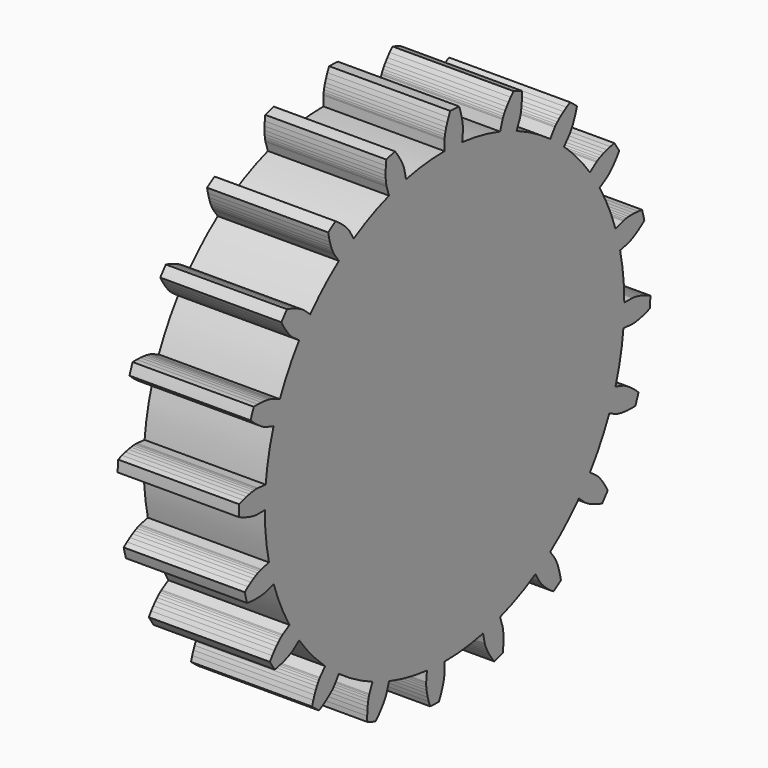
from build123d import *

# Parameters (mm, degrees)
F2_DEPTH = 12.7


# Not quite as in the source:
# - a variable given as a bare number and used for a length is read in inches; the dataset says mm whatever the document's units were


with BuildPart() as f2:
    # F1 (on Right) → F2 (new body)
    with BuildSketch(Plane.YZ):
        with BuildLine():
            ThreePointArc((23.4497989506, -2.3096036071), (23.5348795184, -1.1561944904), (23.5632625, 0))
            ThreePointArc((23.5632625, 0), (23.4259947642, 2.5397064696), (23.0157908626, 5.0498228298))
            ThreePointArc((23.0157908626, 5.0498228298), (22.7402842725, 6.1730714275), (22.4099943458, 7.2814485554))
            ThreePointArc((22.4099943458, 7.2814485554), (21.4946325114, 9.6544348796), (20.3288368046, 11.914937424))
            ThreePointArc((20.3288368046, 11.914937424), (19.7197115612, 12.8980741038), (19.0630798054, 13.8501381934))
            ThreePointArc((19.0630798054, 13.8501381934), (17.4592258664, 15.8241199373), (15.6519545608, 17.6137349268))
            ThreePointArc((15.6519545608, 17.6137349268), (14.7688360869, 18.3605234207), (13.8501381934, 19.0630798054))
            ThreePointArc((13.8501381934, 19.0630798054), (11.7147885481, 20.4448298823), (9.442949951, 21.5883773329))
            ThreePointArc((9.442949951, 21.5883773329), (8.372284036, 22.0257167798), (7.2814485554, 22.4099943458))
            ThreePointArc((7.2814485554, 22.4099943458), (4.8236261049, 23.064257431), (2.3096036071, 23.4497989506))
            ThreePointArc((2.3096036071, 23.4497989506), (1.1561944904, 23.5348795184), (0, 23.5632625))
            ThreePointArc((0, 23.5632625), (-2.5397064696, 23.4259947642), (-5.0498228298, 23.0157908626))
            ThreePointArc((-5.0498228298, 23.0157908626), (-6.1730714275, 22.7402842725), (-7.2814485554, 22.4099943458))
            ThreePointArc((-7.2814485554, 22.4099943458), (-9.6544348796, 21.4946325114), (-11.914937424, 20.3288368046))
            ThreePointArc((-11.914937424, 20.3288368046), (-12.8980741038, 19.7197115612), (-13.8501381934, 19.0630798054))
            ThreePointArc((-13.8501381934, 19.0630798054), (-15.8241199373, 17.4592258664), (-17.6137349268, 15.6519545608))
            ThreePointArc((-17.6137349268, 15.6519545608), (-18.3605234207, 14.7688360869), (-19.0630798054, 13.8501381934))
            ThreePointArc((-19.0630798054, 13.8501381934), (-20.4448298823, 11.7147885481), (-21.5883773329, 9.442949951))
            ThreePointArc((-21.5883773329, 9.442949951), (-22.0257167798, 8.372284036), (-22.4099943458, 7.2814485554))
            ThreePointArc((-22.4099943458, 7.2814485554), (-23.064257431, 4.8236261049), (-23.4497989506, 2.3096036071))
            ThreePointArc((-23.4497989506, 2.3096036071), (-23.5348795184, 1.1561944904), (-23.5632625, 0))
            ThreePointArc((-23.5632625, 0), (-23.4259947642, -2.5397064696), (-23.0157908626, -5.0498228298))
            ThreePointArc((-23.0157908626, -5.0498228298), (-22.7402842725, -6.1730714275), (-22.4099943458, -7.2814485554))
            ThreePointArc((-22.4099943458, -7.2814485554), (-21.4946325114, -9.6544348796), (-20.3288368046, -11.914937424))
            ThreePointArc((-20.3288368046, -11.914937424), (-19.7197115612, -12.8980741038), (-19.0630798054, -13.8501381934))
            ThreePointArc((-19.0630798054, -13.8501381934), (-17.4592258664, -15.8241199373), (-15.6519545608, -17.6137349268))
            ThreePointArc((-15.6519545608, -17.6137349268), (-14.7688360869, -18.3605234207), (-13.8501381934, -19.0630798054))
            ThreePointArc((-13.8501381934, -19.0630798054), (-11.7147885481, -20.4448298823), (-9.442949951, -21.5883773329))
            ThreePointArc((-9.442949951, -21.5883773329), (-8.372284036, -22.0257167798), (-7.2814485554, -22.4099943458))
            ThreePointArc((-7.2814485554, -22.4099943458), (-4.8236261049, -23.064257431), (-2.3096036071, -23.4497989506))
            ThreePointArc((-2.3096036071, -23.4497989506), (-1.1561944904, -23.5348795184), (0, -23.5632625))
            ThreePointArc((0, -23.5632625), (2.5397064696, -23.4259947642), (5.0498228298, -23.0157908626))
            ThreePointArc((5.0498228298, -23.0157908626), (6.1730714275, -22.7402842725), (7.2814485554, -22.4099943458))
            ThreePointArc((7.2814485554, -22.4099943458), (9.6544348796, -21.4946325114), (11.914937424, -20.3288368046))
            ThreePointArc((11.914937424, -20.3288368046), (12.8980741038, -19.7197115612), (13.8501381934, -19.0630798054))
            ThreePointArc((13.8501381934, -19.0630798054), (15.8241199373, -17.4592258664), (17.6137349268, -15.6519545608))
            ThreePointArc((17.6137349268, -15.6519545608), (18.3605234207, -14.7688360869), (19.0630798054, -13.8501381934))
            ThreePointArc((19.0630798054, -13.8501381934), (20.4448298823, -11.7147885481), (21.5883773329, -9.442949951))
            ThreePointArc((21.5883773329, -9.442949951), (22.0257167798, -8.372284036), (22.4099943458, -7.2814485554))
            ThreePointArc((22.4099943458, -7.2814485554), (23.064257431, -4.8236261049), (23.4497989506, -2.3096036071))
        make_face()
        with BuildLine():
            Line((-23.3873833018, -7.5990214781), (-22.4099943458, -7.2814485554))
            ThreePointArc((-22.4099943458, -7.2814485554), (-22.7402842725, -6.1730714275), (-23.0157908626, -5.0498228298))
            Line((-23.0157908626, -5.0498228298), (-24.0196010133, -5.2700656816))
            Line((-24.0196010133, -5.2700656816), (-24.0493872246, -5.2776496958))
            Line((-24.0493872246, -5.2776496958), (-24.1376440155, -5.3043486651))
            Line((-24.1376440155, -5.3043486651), (-24.2823879504, -5.3559820874))
            Line((-24.2823879504, -5.3559820874), (-24.4812024195, -5.4382116757))
            Line((-24.4812024195, -5.4382116757), (-24.7312488149, -5.5565127334))
            Line((-24.7312488149, -5.5565127334), (-25.0292794786, -5.7161462693))
            Line((-25.0292794786, -5.7161462693), (-25.3716523755, -5.9221319592))
            Line((-25.3716523755, -5.9221319592), (-25.7543474377, -6.1792220552))
            Line((-25.7543474377, -6.1792220552), (-26.1729845215, -6.491876343))
            Line((-26.1729845215, -6.491876343), (-26.1912910496, -6.5070292303))
            ThreePointArc((-26.1912910496, -6.5070292303), (-26.0449257315, -7.0701485055), (-25.8864547108, -7.6299815699))
            Line((-25.8864547108, -7.6299815699), (-25.8629988703, -7.633797656))
            Line((-25.8629988703, -7.633797656), (-25.3437303169, -7.6918483328))
            Line((-25.3437303169, -7.6918483328), (-24.8835666247, -7.720136219))
            Line((-24.8835666247, -7.720136219), (-24.4840315708, -7.7247237769))
            Line((-24.4840315708, -7.7247237769), (-24.1461903947, -7.7117437148))
            Line((-24.1461903947, -7.7117437148), (-23.8706469692, -7.6873683017))
            Line((-23.8706469692, -7.6873683017), (-23.6575428926, -7.6577785929))
            Line((-23.6575428926, -7.6577785929), (-23.5065585022, -7.6291336838))
            Line((-23.5065585022, -7.6291336838), (-23.4169158032, -7.6075401056))
            Line((-23.4169158032, -7.6075401056), (-23.3873833018, -7.5990214781))
        make_face()
        with BuildLine():
            Line((-19.8944965109, -14.4541977884), (-19.0630798054, -13.8501381934))
            ThreePointArc((-19.0630798054, -13.8501381934), (-19.7197115612, -12.8980741038), (-20.3288368046, -11.914937424))
            Line((-20.3288368046, -11.914937424), (-21.2154582055, -12.434595219))
            Line((-21.2154582055, -12.434595219), (-21.2414429865, -12.4510124906))
            Line((-21.2414429865, -12.4510124906), (-21.3171297473, -12.5036775676))
            Line((-21.3171297473, -12.5036775676), (-21.4388338049, -12.5975122061))
            Line((-21.4388338049, -12.5975122061), (-21.602507261, -12.7371542416))
            Line((-21.602507261, -12.7371542416), (-21.8037584774, -12.9269338189))
            Line((-21.8037584774, -12.9269338189), (-22.0378730067, -13.1708508734))
            Line((-22.0378730067, -13.1708508734), (-22.2998359026, -13.4725539495))
            Line((-22.2998359026, -13.4725539495), (-22.5843553265, -13.8353204385))
            Line((-22.5843553265, -13.8353204385), (-22.8858873647, -14.2620383097))
            Line((-22.8858873647, -14.2620383097), (-22.8986154078, -14.2821065902))
            ThreePointArc((-22.8986154078, -14.2821065902), (-22.5854002924, -14.7724354756), (-22.2616874646, -15.2558981211))
            Line((-22.2616874646, -15.255898121), (-22.2382003992, -15.2522791813))
            Line((-22.2382003992, -15.2522791813), (-21.7264080121, -15.147025848))
            Line((-21.7264080121, -15.147025848), (-21.2800248965, -15.0317308255))
            Line((-21.2800248965, -15.0317308255), (-20.8986268467, -14.9126307308))
            Line((-20.8986268467, -14.9126307308), (-20.5813318544, -14.7958872934))
            Line((-20.5813318544, -14.7958872934), (-20.326806901, -14.6875572967))
            Line((-20.326806901, -14.6875572967), (-20.1332766032, -14.5935630301))
            Line((-20.1332766032, -14.5935630301), (-19.9985336785, -14.5196633601))
            Line((-19.9985336785, -14.5196633601), (-19.9199511881, -14.4714255295))
            Line((-19.9199511881, -14.4714255295), (-19.8944965109, -14.4541977884))
        make_face()
        with BuildLine():
            Line((-14.4541977884, -19.8944965109), (-13.8501381934, -19.0630798054))
            ThreePointArc((-13.8501381934, -19.0630798054), (-14.7688360869, -18.3605234207), (-15.6519545608, -17.6137349268))
            Line((-15.6519545608, -17.6137349268), (-16.3345985316, -18.3819399395))
            Line((-16.3345985316, -18.3819399395), (-16.3542383111, -18.4055834316))
            Line((-16.3542383111, -18.4055834316), (-16.4099462943, -18.4790593916))
            Line((-16.4099462943, -18.4790593916), (-16.4966972334, -18.605910058))
            Line((-16.4966972334, -18.605910058), (-16.6092081783, -18.7892954052))
            Line((-16.6092081783, -18.7892954052), (-16.7419643445, -19.031976555))
            Line((-16.7419643445, -19.031976555), (-16.8892459781, -19.3363008272))
            Line((-16.8892459781, -19.3363008272), (-17.0451561195, -19.7041884905))
            Line((-17.0451561195, -19.7041884905), (-17.2036491615, -20.137121261))
            Line((-17.2036491615, -20.137121261), (-17.3585600973, -20.6361325971))
            Line((-17.3585600973, -20.6361325971), (-17.3644637459, -20.6591518477))
            ThreePointArc((-17.3644637459, -20.6591518477), (-16.915058511, -21.0286935358), (-16.457791143, -21.38846107))
            Line((-16.457791143, -21.38846107), (-16.4365719304, -21.3777613514))
            Line((-16.4365719304, -21.3777613514), (-15.9823535143, -21.1195069377))
            Line((-15.9823535143, -21.1195069377), (-15.5934460648, -20.8719148865))
            Line((-15.5934460648, -20.8719148865), (-15.2675189175, -20.6407854863))
            Line((-15.2675189175, -20.6407854863), (-15.0018291537, -20.4317063346))
            Line((-15.0018291537, -20.4317063346), (-14.7932373481, -20.2500258493))
            Line((-14.7932373481, -20.2500258493), (-14.6382249231, -20.1008278386))
            Line((-14.6382249231, -20.1008278386), (-14.5329130404, -19.9889072223))
            Line((-14.5329130404, -19.9889072223), (-14.4730829603, -19.9187469941))
            Line((-14.4730829603, -19.9187469941), (-14.4541977884, -19.8944965109))
        make_face()
        with BuildLine():
            Line((-7.5990214781, -23.3873833018), (-7.2814485554, -22.4099943458))
            ThreePointArc((-7.2814485554, -22.4099943458), (-8.372284036, -22.0257167798), (-9.442949951, -21.5883773329))
            Line((-9.442949951, -21.5883773329), (-9.8547945437, -22.5299323042))
            Line((-9.8547945437, -22.5299323042), (-9.866166843, -22.558487627))
            Line((-9.866166843, -22.558487627), (-9.8964429632, -22.6455821311))
            Line((-9.8964429632, -22.6455821311), (-9.9397489974, -22.7930317984))
            Line((-9.9397489974, -22.7930317984), (-9.9900840759, -23.0022094219))
            Line((-9.9900840759, -23.0022094219), (-10.0413500933, -23.2740368222))
            Line((-10.0413500933, -23.2740368222), (-10.0873818788, -23.6089789322))
            Line((-10.0873818788, -23.6089789322), (-10.1219776947, -24.0070397749))
            Line((-10.1219776947, -24.0070397749), (-10.1389299516, -24.4677603508))
            Line((-10.1389299516, -24.4677603508), (-10.1320560234, -24.9902184456))
            Line((-10.1320560234, -24.9902184456), (-10.1305573872, -25.0139353816))
            ThreePointArc((-10.1305573872, -25.0139353816), (-9.5889529483, -25.2265165571), (-9.0428915563, -25.4273724272))
            Line((-9.0428915563, -25.4273724272), (-9.0260172807, -25.4106392928))
            Line((-9.0260172807, -25.4106392928), (-8.6738348989, -25.0246635401))
            Line((-8.6738348989, -25.0246635401), (-8.3804720864, -24.6690104953))
            Line((-8.3804720864, -24.6690104953), (-8.1419198617, -24.3484763457))
            Line((-8.1419198617, -24.3484763457), (-7.9538428915, -24.0675276037))
            Line((-7.9538428915, -24.0675276037), (-7.8116026531, -23.8302807815))
            Line((-7.8116026531, -23.8302807815), (-7.710281797, -23.6404835675))
            Line((-7.710281797, -23.6404835675), (-7.6447096172, -23.5014975746))
            Line((-7.6447096172, -23.5014975746), (-7.6094885324, -23.4162827209))
            Line((-7.6094885324, -23.4162827209), (-7.5990214781, -23.3873833018))
        make_face()
        with BuildLine():
            Line((0, -24.5909500656), (0, -23.5632625))
            ThreePointArc((0, -23.5632625), (-1.1561944904, -23.5348795184), (-2.3096036071, -23.4497989506))
            Line((-2.3096036071, -23.4497989506), (-2.4103346034, -24.4725379196))
            Line((-2.4103346034, -24.4725379196), (-2.4123262228, -24.5032098793))
            Line((-2.4123262228, -24.5032098793), (-2.4142068423, -24.5953975106))
            Line((-2.4142068423, -24.5953975106), (-2.4098288753, -24.749012778))
            Line((-2.4098288753, -24.749012778), (-2.3930609392, -24.9635069146))
            Line((-2.3930609392, -24.9635069146), (-2.3578185329, -25.2378722056))
            Line((-2.3578185329, -25.2378722056), (-2.2980945583, -25.5706456859))
            Line((-2.2980945583, -25.5706456859), (-2.2079895693, -25.9599147393))
            Line((-2.2079895693, -25.9599147393), (-2.0817416361, -26.4033245806))
            Line((-2.0817416361, -26.4033245806), (-1.9137557117, -26.8980875955))
            Line((-1.9137557117, -26.8980875955), (-1.9050014877, -26.920180638))
            ThreePointArc((-1.9050014877, -26.920180638), (-1.3242138609, -26.9549923743), (-0.7428107384, -26.9772754083))
            Line((-0.7428107384, -26.9772754083), (-0.7319331716, -26.9561468139))
            Line((-0.7319331716, -26.9561468139), (-0.5162608895, -26.4802317181))
            Line((-0.5162608895, -26.4802317181), (-0.3471591099, -26.0513314777))
            Line((-0.3471591099, -26.0513314777), (-0.2193329616, -25.6727686945))
            Line((-0.2193329616, -25.6727686945), (-0.1272790694, -25.3474515827))
            Line((-0.1272790694, -25.3474515827), (-0.0653138637, -25.0778617955))
            Line((-0.0653138637, -25.0778617955), (-0.0276025679, -24.8660440519))
            Line((-0.0276025679, -24.8660440519), (-0.0081887528, -24.7135975998))
            Line((-0.0081887528, -24.7135975998), (-0.0010243486, -24.6216695442))
            Line((-0.0010243486, -24.6216695442), (0, -24.5909500656))
        make_face()
        with BuildLine():
            Line((7.5990214781, -23.3873833018), (7.2814485554, -22.4099943458))
            ThreePointArc((7.2814485554, -22.4099943458), (6.1730714275, -22.7402842725), (5.0498228298, -23.0157908626))
            Line((5.0498228298, -23.0157908626), (5.2700656816, -24.0196010133))
            Line((5.2700656816, -24.0196010133), (5.2776496958, -24.0493872246))
            Line((5.2776496958, -24.0493872246), (5.3043486651, -24.1376440155))
            Line((5.3043486651, -24.1376440155), (5.3559820874, -24.2823879504))
            Line((5.3559820874, -24.2823879504), (5.4382116757, -24.4812024195))
            Line((5.4382116757, -24.4812024195), (5.5565127334, -24.7312488149))
            Line((5.5565127334, -24.7312488149), (5.7161462693, -25.0292794786))
            Line((5.7161462693, -25.0292794786), (5.9221319592, -25.3716523755))
            Line((5.9221319592, -25.3716523755), (6.1792220552, -25.7543474377))
            Line((6.1792220552, -25.7543474377), (6.491876343, -26.1729845215))
            Line((6.491876343, -26.1729845215), (6.5070292303, -26.1912910496))
            ThreePointArc((6.5070292303, -26.1912910496), (7.0701485055, -26.0449257315), (7.6299815699, -25.8864547108))
            Line((7.6299815699, -25.8864547108), (7.633797656, -25.8629988703))
            Line((7.633797656, -25.8629988703), (7.6918483328, -25.3437303169))
            Line((7.6918483328, -25.3437303169), (7.720136219, -24.8835666247))
            Line((7.720136219, -24.8835666247), (7.7247237769, -24.4840315708))
            Line((7.7247237769, -24.4840315708), (7.7117437148, -24.1461903947))
            Line((7.7117437148, -24.1461903947), (7.6873683017, -23.8706469692))
            Line((7.6873683017, -23.8706469692), (7.6577785929, -23.6575428926))
            Line((7.6577785929, -23.6575428926), (7.6291336838, -23.5065585022))
            Line((7.6291336838, -23.5065585022), (7.6075401056, -23.4169158032))
            Line((7.6075401056, -23.4169158032), (7.5990214781, -23.3873833018))
        make_face()
        with BuildLine():
            Line((14.4541977884, -19.8944965109), (13.8501381934, -19.0630798054))
            ThreePointArc((13.8501381934, -19.0630798054), (12.8980741038, -19.7197115612), (11.914937424, -20.3288368046))
            Line((11.914937424, -20.3288368046), (12.434595219, -21.2154582055))
            Line((12.434595219, -21.2154582055), (12.4510124906, -21.2414429865))
            Line((12.4510124906, -21.2414429865), (12.5036775676, -21.3171297473))
            Line((12.5036775676, -21.3171297473), (12.5975122061, -21.4388338049))
            Line((12.5975122061, -21.4388338049), (12.7371542416, -21.602507261))
            Line((12.7371542416, -21.602507261), (12.9269338189, -21.8037584774))
            Line((12.9269338189, -21.8037584774), (13.1708508734, -22.0378730067))
            Line((13.1708508734, -22.0378730067), (13.4725539495, -22.2998359026))
            Line((13.4725539495, -22.2998359026), (13.8353204385, -22.5843553265))
            Line((13.8353204385, -22.5843553265), (14.2620383097, -22.8858873647))
            Line((14.2620383097, -22.8858873647), (14.2821065902, -22.8986154078))
            ThreePointArc((14.2821065902, -22.8986154078), (14.7724354756, -22.5854002924), (15.2558981211, -22.2616874646))
            Line((15.255898121, -22.2616874646), (15.2522791813, -22.2382003992))
            Line((15.2522791813, -22.2382003992), (15.147025848, -21.7264080121))
            Line((15.147025848, -21.7264080121), (15.0317308255, -21.2800248965))
            Line((15.0317308255, -21.2800248965), (14.9126307308, -20.8986268467))
            Line((14.9126307308, -20.8986268467), (14.7958872934, -20.5813318544))
            Line((14.7958872934, -20.5813318544), (14.6875572967, -20.326806901))
            Line((14.6875572967, -20.326806901), (14.5935630301, -20.1332766032))
            Line((14.5935630301, -20.1332766032), (14.5196633601, -19.9985336785))
            Line((14.5196633601, -19.9985336785), (14.4714255295, -19.9199511881))
            Line((14.4714255295, -19.9199511881), (14.4541977884, -19.8944965109))
        make_face()
        with BuildLine():
            Line((19.8944965109, -14.4541977884), (19.0630798054, -13.8501381934))
            ThreePointArc((19.0630798054, -13.8501381934), (18.3605234207, -14.7688360869), (17.6137349268, -15.6519545608))
            Line((17.6137349268, -15.6519545608), (18.3819399395, -16.3345985316))
            Line((18.3819399395, -16.3345985316), (18.4055834316, -16.3542383111))
            Line((18.4055834316, -16.3542383111), (18.4790593916, -16.4099462943))
            Line((18.4790593916, -16.4099462943), (18.605910058, -16.4966972334))
            Line((18.605910058, -16.4966972334), (18.7892954052, -16.6092081783))
            Line((18.7892954052, -16.6092081783), (19.031976555, -16.7419643445))
            Line((19.031976555, -16.7419643445), (19.3363008272, -16.8892459781))
            Line((19.3363008272, -16.8892459781), (19.7041884905, -17.0451561195))
            Line((19.7041884905, -17.0451561195), (20.137121261, -17.2036491615))
            Line((20.137121261, -17.2036491615), (20.6361325971, -17.3585600973))
            Line((20.6361325971, -17.3585600973), (20.6591518477, -17.3644637459))
            ThreePointArc((20.6591518477, -17.3644637459), (21.0286935358, -16.915058511), (21.38846107, -16.457791143))
            Line((21.38846107, -16.457791143), (21.3777613514, -16.4365719304))
            Line((21.3777613514, -16.4365719304), (21.1195069377, -15.9823535143))
            Line((21.1195069377, -15.9823535143), (20.8719148865, -15.5934460648))
            Line((20.8719148865, -15.5934460648), (20.6407854863, -15.2675189175))
            Line((20.6407854863, -15.2675189175), (20.4317063346, -15.0018291537))
            Line((20.4317063346, -15.0018291537), (20.2500258493, -14.7932373481))
            Line((20.2500258493, -14.7932373481), (20.1008278386, -14.6382249231))
            Line((20.1008278386, -14.6382249231), (19.9889072223, -14.5329130404))
            Line((19.9889072223, -14.5329130404), (19.9187469941, -14.4730829603))
            Line((19.9187469941, -14.4730829603), (19.8944965109, -14.4541977884))
        make_face()
        with BuildLine():
            Line((23.3873833018, -7.5990214781), (22.4099943458, -7.2814485554))
            ThreePointArc((22.4099943458, -7.2814485554), (22.0257167798, -8.372284036), (21.5883773329, -9.442949951))
            Line((21.5883773329, -9.442949951), (22.5299323042, -9.8547945437))
            Line((22.5299323042, -9.8547945437), (22.558487627, -9.866166843))
            Line((22.558487627, -9.866166843), (22.6455821311, -9.8964429632))
            Line((22.6455821311, -9.8964429632), (22.7930317984, -9.9397489974))
            Line((22.7930317984, -9.9397489974), (23.0022094219, -9.9900840759))
            Line((23.0022094219, -9.9900840759), (23.2740368222, -10.0413500933))
            Line((23.2740368222, -10.0413500933), (23.6089789322, -10.0873818788))
            Line((23.6089789322, -10.0873818788), (24.0070397749, -10.1219776947))
            Line((24.0070397749, -10.1219776947), (24.4677603508, -10.1389299516))
            Line((24.4677603508, -10.1389299516), (24.9902184456, -10.1320560234))
            Line((24.9902184456, -10.1320560234), (25.0139353816, -10.1305573872))
            ThreePointArc((25.0139353816, -10.1305573872), (25.2265165571, -9.5889529483), (25.4273724272, -9.0428915563))
            Line((25.4273724272, -9.0428915563), (25.4106392928, -9.0260172807))
            Line((25.4106392928, -9.0260172807), (25.0246635401, -8.6738348989))
            Line((25.0246635401, -8.6738348989), (24.6690104953, -8.3804720864))
            Line((24.6690104953, -8.3804720864), (24.3484763457, -8.1419198617))
            Line((24.3484763457, -8.1419198617), (24.0675276037, -7.9538428915))
            Line((24.0675276037, -7.9538428915), (23.8302807815, -7.8116026531))
            Line((23.8302807815, -7.8116026531), (23.6404835675, -7.710281797))
            Line((23.6404835675, -7.710281797), (23.5014975746, -7.6447096172))
            Line((23.5014975746, -7.6447096172), (23.4162827209, -7.6094885324))
            Line((23.4162827209, -7.6094885324), (23.3873833018, -7.5990214781))
        make_face()
        with BuildLine():
            Line((24.5909500656, 0), (23.5632625, 0))
            ThreePointArc((23.5632625, 0), (23.5348795184, -1.1561944904), (23.4497989506, -2.3096036071))
            Line((23.4497989506, -2.3096036071), (24.4725379196, -2.4103346034))
            Line((24.4725379196, -2.4103346034), (24.5032098793, -2.4123262228))
            Line((24.5032098793, -2.4123262228), (24.5953975106, -2.4142068423))
            Line((24.5953975106, -2.4142068423), (24.749012778, -2.4098288753))
            Line((24.749012778, -2.4098288753), (24.9635069146, -2.3930609392))
            Line((24.9635069146, -2.3930609392), (25.2378722056, -2.3578185329))
            Line((25.2378722056, -2.3578185329), (25.5706456859, -2.2980945583))
            Line((25.5706456859, -2.2980945583), (25.9599147393, -2.2079895693))
            Line((25.9599147393, -2.2079895693), (26.4033245806, -2.0817416361))
            Line((26.4033245806, -2.0817416361), (26.8980875955, -1.9137557117))
            Line((26.8980875955, -1.9137557117), (26.920180638, -1.9050014877))
            ThreePointArc((26.920180638, -1.9050014877), (26.9549923743, -1.3242138609), (26.9772754083, -0.7428107384))
            Line((26.9772754083, -0.7428107384), (26.9561468139, -0.7319331716))
            Line((26.9561468139, -0.7319331716), (26.4802317181, -0.5162608895))
            Line((26.4802317181, -0.5162608895), (26.0513314777, -0.3471591099))
            Line((26.0513314777, -0.3471591099), (25.6727686945, -0.2193329616))
            Line((25.6727686945, -0.2193329616), (25.3474515827, -0.1272790694))
            Line((25.3474515827, -0.1272790694), (25.0778617955, -0.0653138637))
            Line((25.0778617955, -0.0653138637), (24.8660440519, -0.0276025679))
            Line((24.8660440519, -0.0276025679), (24.7135975998, -0.0081887528))
            Line((24.7135975998, -0.0081887528), (24.6216695442, -0.0010243486))
            Line((24.6216695442, -0.0010243486), (24.5909500656, 0))
        make_face()
        with BuildLine():
            ThreePointArc((22.4099943458, 7.2814485554), (22.7402842725, 6.1730714275), (23.0157908626, 5.0498228298))
            Line((23.0157908626, 5.0498228298), (24.0196010133, 5.2700656816))
            Line((24.0196010133, 5.2700656816), (24.0493872246, 5.2776496958))
            Line((24.0493872246, 5.2776496958), (24.1376440155, 5.3043486651))
            Line((24.1376440155, 5.3043486651), (24.2823879504, 5.3559820874))
            Line((24.2823879504, 5.3559820874), (24.4812024195, 5.4382116757))
            Line((24.4812024195, 5.4382116757), (24.7312488149, 5.5565127334))
            Line((24.7312488149, 5.5565127334), (25.0292794786, 5.7161462693))
            Line((25.0292794786, 5.7161462693), (25.3716523755, 5.9221319592))
            Line((25.3716523755, 5.9221319592), (25.7543474377, 6.1792220552))
            Line((25.7543474377, 6.1792220552), (26.1729845215, 6.491876343))
            Line((26.1729845215, 6.491876343), (26.1912910496, 6.5070292303))
            ThreePointArc((26.1912910496, 6.5070292303), (26.0449257315, 7.0701485055), (25.8864547108, 7.6299815699))
            Line((25.8864547108, 7.6299815699), (25.8629988703, 7.633797656))
            Line((25.8629988703, 7.633797656), (25.3437303169, 7.6918483328))
            Line((25.3437303169, 7.6918483328), (24.8835666247, 7.720136219))
            Line((24.8835666247, 7.720136219), (24.4840315708, 7.7247237769))
            Line((24.4840315708, 7.7247237769), (24.1461903947, 7.7117437148))
            Line((24.1461903947, 7.7117437148), (23.8706469692, 7.6873683017))
            Line((23.8706469692, 7.6873683017), (23.6575428926, 7.6577785929))
            Line((23.6575428926, 7.6577785929), (23.5065585022, 7.6291336838))
            Line((23.5065585022, 7.6291336838), (23.4169158032, 7.6075401056))
            Line((23.4169158032, 7.6075401056), (23.3873833018, 7.5990214781))
            Line((23.3873833018, 7.5990214781), (22.4099943458, 7.2814485554))
        make_face()
        with BuildLine():
            ThreePointArc((19.0630798054, 13.8501381934), (19.7197115612, 12.8980741038), (20.3288368046, 11.914937424))
            Line((20.3288368046, 11.914937424), (21.2154582055, 12.434595219))
            Line((21.2154582055, 12.434595219), (21.2414429865, 12.4510124906))
            Line((21.2414429865, 12.4510124906), (21.3171297473, 12.5036775676))
            Line((21.3171297473, 12.5036775676), (21.4388338049, 12.5975122061))
            Line((21.4388338049, 12.5975122061), (21.602507261, 12.7371542416))
            Line((21.602507261, 12.7371542416), (21.8037584774, 12.9269338189))
            Line((21.8037584774, 12.9269338189), (22.0378730067, 13.1708508734))
            Line((22.0378730067, 13.1708508734), (22.2998359026, 13.4725539495))
            Line((22.2998359026, 13.4725539495), (22.5843553265, 13.8353204385))
            Line((22.5843553265, 13.8353204385), (22.8858873647, 14.2620383097))
            Line((22.8858873647, 14.2620383097), (22.8986154078, 14.2821065902))
            ThreePointArc((22.8986154078, 14.2821065902), (22.5854002924, 14.7724354756), (22.2616874646, 15.2558981211))
            Line((22.2616874646, 15.255898121), (22.2382003992, 15.2522791813))
            Line((22.2382003992, 15.2522791813), (21.7264080121, 15.147025848))
            Line((21.7264080121, 15.147025848), (21.2800248965, 15.0317308255))
            Line((21.2800248965, 15.0317308255), (20.8986268467, 14.9126307308))
            Line((20.8986268467, 14.9126307308), (20.5813318544, 14.7958872934))
            Line((20.5813318544, 14.7958872934), (20.326806901, 14.6875572967))
            Line((20.326806901, 14.6875572967), (20.1332766032, 14.5935630301))
            Line((20.1332766032, 14.5935630301), (19.9985336785, 14.5196633601))
            Line((19.9985336785, 14.5196633601), (19.9199511881, 14.4714255295))
            Line((19.9199511881, 14.4714255295), (19.8944965109, 14.4541977884))
            Line((19.8944965109, 14.4541977884), (19.0630798054, 13.8501381934))
        make_face()
        with BuildLine():
            ThreePointArc((13.8501381934, 19.0630798054), (14.7688360869, 18.3605234207), (15.6519545608, 17.6137349268))
            Line((15.6519545608, 17.6137349268), (16.3345985316, 18.3819399395))
            Line((16.3345985316, 18.3819399395), (16.3542383111, 18.4055834316))
            Line((16.3542383111, 18.4055834316), (16.4099462943, 18.4790593916))
            Line((16.4099462943, 18.4790593916), (16.4966972334, 18.605910058))
            Line((16.4966972334, 18.605910058), (16.6092081783, 18.7892954052))
            Line((16.6092081783, 18.7892954052), (16.7419643445, 19.031976555))
            Line((16.7419643445, 19.031976555), (16.8892459781, 19.3363008272))
            Line((16.8892459781, 19.3363008272), (17.0451561195, 19.7041884905))
            Line((17.0451561195, 19.7041884905), (17.2036491615, 20.137121261))
            Line((17.2036491615, 20.137121261), (17.3585600973, 20.6361325971))
            Line((17.3585600973, 20.6361325971), (17.3644637459, 20.6591518477))
            ThreePointArc((17.3644637459, 20.6591518477), (16.915058511, 21.0286935358), (16.457791143, 21.38846107))
            Line((16.457791143, 21.38846107), (16.4365719304, 21.3777613514))
            Line((16.4365719304, 21.3777613514), (15.9823535143, 21.1195069377))
            Line((15.9823535143, 21.1195069377), (15.5934460648, 20.8719148865))
            Line((15.5934460648, 20.8719148865), (15.2675189175, 20.6407854863))
            Line((15.2675189175, 20.6407854863), (15.0018291537, 20.4317063346))
            Line((15.0018291537, 20.4317063346), (14.7932373481, 20.2500258493))
            Line((14.7932373481, 20.2500258493), (14.6382249231, 20.1008278386))
            Line((14.6382249231, 20.1008278386), (14.5329130404, 19.9889072223))
            Line((14.5329130404, 19.9889072223), (14.4730829603, 19.9187469941))
            Line((14.4730829603, 19.9187469941), (14.4541977884, 19.8944965109))
            Line((14.4541977884, 19.8944965109), (13.8501381934, 19.0630798054))
        make_face()
        with BuildLine():
            ThreePointArc((7.2814485554, 22.4099943458), (8.372284036, 22.0257167798), (9.442949951, 21.5883773329))
            Line((9.442949951, 21.5883773329), (9.8547945437, 22.5299323042))
            Line((9.8547945437, 22.5299323042), (9.866166843, 22.558487627))
            Line((9.866166843, 22.558487627), (9.8964429632, 22.6455821311))
            Line((9.8964429632, 22.6455821311), (9.9397489974, 22.7930317984))
            Line((9.9397489974, 22.7930317984), (9.9900840759, 23.0022094219))
            Line((9.9900840759, 23.0022094219), (10.0413500933, 23.2740368222))
            Line((10.0413500933, 23.2740368222), (10.0873818788, 23.6089789322))
            Line((10.0873818788, 23.6089789322), (10.1219776947, 24.0070397749))
            Line((10.1219776947, 24.0070397749), (10.1389299516, 24.4677603508))
            Line((10.1389299516, 24.4677603508), (10.1320560234, 24.9902184456))
            Line((10.1320560234, 24.9902184456), (10.1305573872, 25.0139353816))
            ThreePointArc((10.1305573872, 25.0139353816), (9.5889529483, 25.2265165571), (9.0428915563, 25.4273724272))
            Line((9.0428915563, 25.4273724272), (9.0260172807, 25.4106392928))
            Line((9.0260172807, 25.4106392928), (8.6738348989, 25.0246635401))
            Line((8.6738348989, 25.0246635401), (8.3804720864, 24.6690104953))
            Line((8.3804720864, 24.6690104953), (8.1419198617, 24.3484763457))
            Line((8.1419198617, 24.3484763457), (7.9538428915, 24.0675276037))
            Line((7.9538428915, 24.0675276037), (7.8116026531, 23.8302807815))
            Line((7.8116026531, 23.8302807815), (7.710281797, 23.6404835675))
            Line((7.710281797, 23.6404835675), (7.6447096172, 23.5014975746))
            Line((7.6447096172, 23.5014975746), (7.6094885324, 23.4162827209))
            Line((7.6094885324, 23.4162827209), (7.5990214781, 23.3873833018))
            Line((7.5990214781, 23.3873833018), (7.2814485554, 22.4099943458))
        make_face()
        with BuildLine():
            ThreePointArc((0, 23.5632625), (1.1561944904, 23.5348795184), (2.3096036071, 23.4497989506))
            Line((2.3096036071, 23.4497989506), (2.4103346034, 24.4725379196))
            Line((2.4103346034, 24.4725379196), (2.4123262228, 24.5032098793))
            Line((2.4123262228, 24.5032098793), (2.4142068423, 24.5953975106))
            Line((2.4142068423, 24.5953975106), (2.4098288753, 24.749012778))
            Line((2.4098288753, 24.749012778), (2.3930609392, 24.9635069146))
            Line((2.3930609392, 24.9635069146), (2.3578185329, 25.2378722056))
            Line((2.3578185329, 25.2378722056), (2.2980945583, 25.5706456859))
            Line((2.2980945583, 25.5706456859), (2.2079895693, 25.9599147393))
            Line((2.2079895693, 25.9599147393), (2.0817416361, 26.4033245806))
            Line((2.0817416361, 26.4033245806), (1.9137557117, 26.8980875955))
            Line((1.9137557117, 26.8980875955), (1.9050014877, 26.920180638))
            ThreePointArc((1.9050014877, 26.920180638), (1.3242138609, 26.9549923743), (0.7428107384, 26.9772754083))
            Line((0.7428107384, 26.9772754083), (0.7319331716, 26.9561468139))
            Line((0.7319331716, 26.9561468139), (0.5162608895, 26.4802317181))
            Line((0.5162608895, 26.4802317181), (0.3471591099, 26.0513314777))
            Line((0.3471591099, 26.0513314777), (0.2193329616, 25.6727686945))
            Line((0.2193329616, 25.6727686945), (0.1272790694, 25.3474515827))
            Line((0.1272790694, 25.3474515827), (0.0653138637, 25.0778617955))
            Line((0.0653138637, 25.0778617955), (0.0276025679, 24.8660440519))
            Line((0.0276025679, 24.8660440519), (0.0081887528, 24.7135975998))
            Line((0.0081887528, 24.7135975998), (0.0010243486, 24.6216695442))
            Line((0.0010243486, 24.6216695442), (0, 24.5909500656))
            Line((0, 24.5909500656), (0, 23.5632625))
        make_face()
        with BuildLine():
            ThreePointArc((-7.2814485554, 22.4099943458), (-6.1730714275, 22.7402842725), (-5.0498228298, 23.0157908626))
            Line((-5.0498228298, 23.0157908626), (-5.2700656816, 24.0196010133))
            Line((-5.2700656816, 24.0196010133), (-5.2776496958, 24.0493872246))
            Line((-5.2776496958, 24.0493872246), (-5.3043486651, 24.1376440155))
            Line((-5.3043486651, 24.1376440155), (-5.3559820874, 24.2823879504))
            Line((-5.3559820874, 24.2823879504), (-5.4382116757, 24.4812024195))
            Line((-5.4382116757, 24.4812024195), (-5.5565127334, 24.7312488149))
            Line((-5.5565127334, 24.7312488149), (-5.7161462693, 25.0292794786))
            Line((-5.7161462693, 25.0292794786), (-5.9221319592, 25.3716523755))
            Line((-5.9221319592, 25.3716523755), (-6.1792220552, 25.7543474377))
            Line((-6.1792220552, 25.7543474377), (-6.491876343, 26.1729845215))
            Line((-6.491876343, 26.1729845215), (-6.5070292303, 26.1912910496))
            ThreePointArc((-6.5070292303, 26.1912910496), (-7.0701485055, 26.0449257315), (-7.6299815699, 25.8864547108))
            Line((-7.6299815699, 25.8864547108), (-7.633797656, 25.8629988703))
            Line((-7.633797656, 25.8629988703), (-7.6918483328, 25.3437303169))
            Line((-7.6918483328, 25.3437303169), (-7.720136219, 24.8835666247))
            Line((-7.720136219, 24.8835666247), (-7.7247237769, 24.4840315708))
            Line((-7.7247237769, 24.4840315708), (-7.7117437148, 24.1461903947))
            Line((-7.7117437148, 24.1461903947), (-7.6873683017, 23.8706469692))
            Line((-7.6873683017, 23.8706469692), (-7.6577785929, 23.6575428926))
            Line((-7.6577785929, 23.6575428926), (-7.6291336838, 23.5065585022))
            Line((-7.6291336838, 23.5065585022), (-7.6075401056, 23.4169158032))
            Line((-7.6075401056, 23.4169158032), (-7.5990214781, 23.3873833018))
            Line((-7.5990214781, 23.3873833018), (-7.2814485554, 22.4099943458))
        make_face()
        with BuildLine():
            ThreePointArc((-13.8501381934, 19.0630798054), (-12.8980741038, 19.7197115612), (-11.914937424, 20.3288368046))
            Line((-11.914937424, 20.3288368046), (-12.434595219, 21.2154582055))
            Line((-12.434595219, 21.2154582055), (-12.4510124906, 21.2414429865))
            Line((-12.4510124906, 21.2414429865), (-12.5036775676, 21.3171297473))
            Line((-12.5036775676, 21.3171297473), (-12.5975122061, 21.4388338049))
            Line((-12.5975122061, 21.4388338049), (-12.7371542416, 21.602507261))
            Line((-12.7371542416, 21.602507261), (-12.9269338189, 21.8037584774))
            Line((-12.9269338189, 21.8037584774), (-13.1708508734, 22.0378730067))
            Line((-13.1708508734, 22.0378730067), (-13.4725539495, 22.2998359026))
            Line((-13.4725539495, 22.2998359026), (-13.8353204385, 22.5843553265))
            Line((-13.8353204385, 22.5843553265), (-14.2620383097, 22.8858873647))
            Line((-14.2620383097, 22.8858873647), (-14.2821065902, 22.8986154078))
            ThreePointArc((-14.2821065902, 22.8986154078), (-14.7724354756, 22.5854002924), (-15.2558981211, 22.2616874646))
            Line((-15.255898121, 22.2616874646), (-15.2522791813, 22.2382003992))
            Line((-15.2522791813, 22.2382003992), (-15.147025848, 21.7264080121))
            Line((-15.147025848, 21.7264080121), (-15.0317308255, 21.2800248965))
            Line((-15.0317308255, 21.2800248965), (-14.9126307308, 20.8986268467))
            Line((-14.9126307308, 20.8986268467), (-14.7958872934, 20.5813318544))
            Line((-14.7958872934, 20.5813318544), (-14.6875572967, 20.326806901))
            Line((-14.6875572967, 20.326806901), (-14.5935630301, 20.1332766032))
            Line((-14.5935630301, 20.1332766032), (-14.5196633601, 19.9985336785))
            Line((-14.5196633601, 19.9985336785), (-14.4714255295, 19.9199511881))
            Line((-14.4714255295, 19.9199511881), (-14.4541977884, 19.8944965109))
            Line((-14.4541977884, 19.8944965109), (-13.8501381934, 19.0630798054))
        make_face()
        with BuildLine():
            ThreePointArc((-19.0630798054, 13.8501381934), (-18.3605234207, 14.7688360869), (-17.6137349268, 15.6519545608))
            Line((-17.6137349268, 15.6519545608), (-18.3819399395, 16.3345985316))
            Line((-18.3819399395, 16.3345985316), (-18.4055834316, 16.3542383111))
            Line((-18.4055834316, 16.3542383111), (-18.4790593916, 16.4099462943))
            Line((-18.4790593916, 16.4099462943), (-18.605910058, 16.4966972334))
            Line((-18.605910058, 16.4966972334), (-18.7892954052, 16.6092081783))
            Line((-18.7892954052, 16.6092081783), (-19.031976555, 16.7419643445))
            Line((-19.031976555, 16.7419643445), (-19.3363008272, 16.8892459781))
            Line((-19.3363008272, 16.8892459781), (-19.7041884905, 17.0451561195))
            Line((-19.7041884905, 17.0451561195), (-20.137121261, 17.2036491615))
            Line((-20.137121261, 17.2036491615), (-20.6361325971, 17.3585600973))
            Line((-20.6361325971, 17.3585600973), (-20.6591518477, 17.3644637459))
            ThreePointArc((-20.6591518477, 17.3644637459), (-21.0286935358, 16.915058511), (-21.38846107, 16.457791143))
            Line((-21.38846107, 16.457791143), (-21.3777613514, 16.4365719304))
            Line((-21.3777613514, 16.4365719304), (-21.1195069377, 15.9823535143))
            Line((-21.1195069377, 15.9823535143), (-20.8719148865, 15.5934460648))
            Line((-20.8719148865, 15.5934460648), (-20.6407854863, 15.2675189175))
            Line((-20.6407854863, 15.2675189175), (-20.4317063346, 15.0018291537))
            Line((-20.4317063346, 15.0018291537), (-20.2500258493, 14.7932373481))
            Line((-20.2500258493, 14.7932373481), (-20.1008278386, 14.6382249231))
            Line((-20.1008278386, 14.6382249231), (-19.9889072223, 14.5329130404))
            Line((-19.9889072223, 14.5329130404), (-19.9187469941, 14.4730829603))
            Line((-19.9187469941, 14.4730829603), (-19.8944965109, 14.4541977884))
            Line((-19.8944965109, 14.4541977884), (-19.0630798054, 13.8501381934))
        make_face()
        with BuildLine():
            ThreePointArc((-22.4099943458, 7.2814485554), (-22.0257167798, 8.372284036), (-21.5883773329, 9.442949951))
            Line((-21.5883773329, 9.442949951), (-22.5299323042, 9.8547945437))
            Line((-22.5299323042, 9.8547945437), (-22.558487627, 9.866166843))
            Line((-22.558487627, 9.866166843), (-22.6455821311, 9.8964429632))
            Line((-22.6455821311, 9.8964429632), (-22.7930317984, 9.9397489974))
            Line((-22.7930317984, 9.9397489974), (-23.0022094219, 9.9900840759))
            Line((-23.0022094219, 9.9900840759), (-23.2740368222, 10.0413500933))
            Line((-23.2740368222, 10.0413500933), (-23.6089789322, 10.0873818788))
            Line((-23.6089789322, 10.0873818788), (-24.0070397749, 10.1219776947))
            Line((-24.0070397749, 10.1219776947), (-24.4677603508, 10.1389299516))
            Line((-24.4677603508, 10.1389299516), (-24.9902184456, 10.1320560234))
            Line((-24.9902184456, 10.1320560234), (-25.0139353816, 10.1305573872))
            ThreePointArc((-25.0139353816, 10.1305573872), (-25.2265165571, 9.5889529483), (-25.4273724272, 9.0428915563))
            Line((-25.4273724272, 9.0428915563), (-25.4106392928, 9.0260172807))
            Line((-25.4106392928, 9.0260172807), (-25.0246635401, 8.6738348989))
            Line((-25.0246635401, 8.6738348989), (-24.6690104953, 8.3804720864))
            Line((-24.6690104953, 8.3804720864), (-24.3484763457, 8.1419198617))
            Line((-24.3484763457, 8.1419198617), (-24.0675276037, 7.9538428915))
            Line((-24.0675276037, 7.9538428915), (-23.8302807815, 7.8116026531))
            Line((-23.8302807815, 7.8116026531), (-23.6404835675, 7.710281797))
            Line((-23.6404835675, 7.710281797), (-23.5014975746, 7.6447096172))
            Line((-23.5014975746, 7.6447096172), (-23.4162827209, 7.6094885324))
            Line((-23.4162827209, 7.6094885324), (-23.3873833018, 7.5990214781))
            Line((-23.3873833018, 7.5990214781), (-22.4099943458, 7.2814485554))
        make_face()
        with BuildLine():
            ThreePointArc((-23.5632625, 0), (-23.5348795184, 1.1561944904), (-23.4497989506, 2.3096036071))
            Line((-23.4497989506, 2.3096036071), (-24.4725379196, 2.4103346034))
            Line((-24.4725379196, 2.4103346034), (-24.5032098793, 2.4123262228))
            Line((-24.5032098793, 2.4123262228), (-24.5953975106, 2.4142068423))
            Line((-24.5953975106, 2.4142068423), (-24.749012778, 2.4098288753))
            Line((-24.749012778, 2.4098288753), (-24.9635069146, 2.3930609392))
            Line((-24.9635069146, 2.3930609392), (-25.2378722056, 2.3578185329))
            Line((-25.2378722056, 2.3578185329), (-25.5706456859, 2.2980945583))
            Line((-25.5706456859, 2.2980945583), (-25.9599147393, 2.2079895693))
            Line((-25.9599147393, 2.2079895693), (-26.4033245806, 2.0817416361))
            Line((-26.4033245806, 2.0817416361), (-26.8980875955, 1.9137557117))
            Line((-26.8980875955, 1.9137557117), (-26.920180638, 1.9050014877))
            ThreePointArc((-26.920180638, 1.9050014877), (-26.9549923743, 1.3242138609), (-26.9772754083, 0.7428107384))
            Line((-26.9772754083, 0.7428107384), (-26.9561468139, 0.7319331716))
            Line((-26.9561468139, 0.7319331716), (-26.4802317181, 0.5162608895))
            Line((-26.4802317181, 0.5162608895), (-26.0513314777, 0.3471591099))
            Line((-26.0513314777, 0.3471591099), (-25.6727686945, 0.2193329616))
            Line((-25.6727686945, 0.2193329616), (-25.3474515827, 0.1272790694))
            Line((-25.3474515827, 0.1272790694), (-25.0778617955, 0.0653138637))
            Line((-25.0778617955, 0.0653138637), (-24.8660440519, 0.0276025679))
            Line((-24.8660440519, 0.0276025679), (-24.7135975998, 0.0081887528))
            Line((-24.7135975998, 0.0081887528), (-24.6216695442, 0.0010243486))
            Line((-24.6216695442, 0.0010243486), (-24.5909500656, 0))
            Line((-24.5909500656, 0), (-23.5632625, 0))
        make_face()
    extrude(amount=F2_DEPTH)


solid = f2.part
